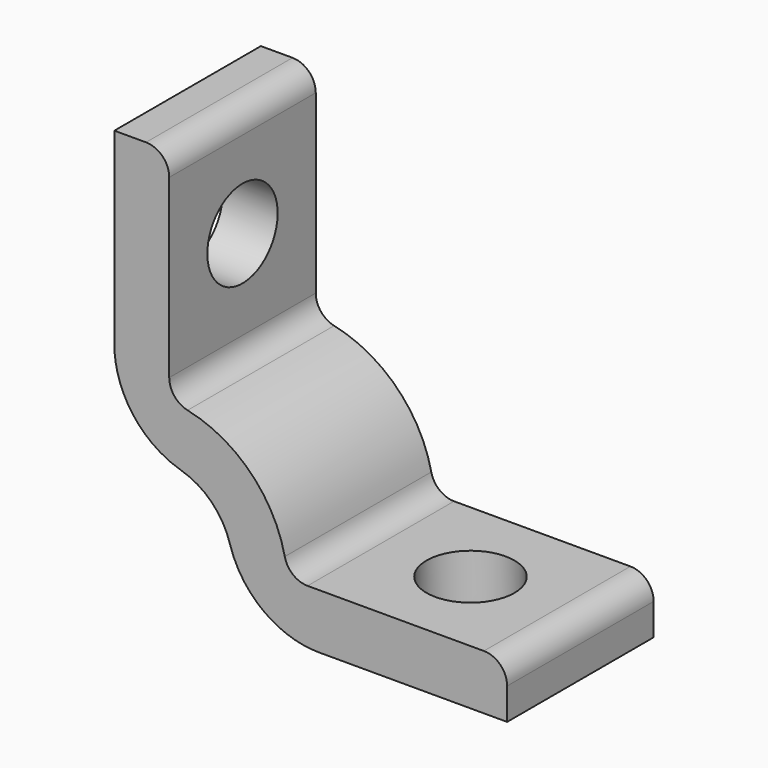
from build123d import *

# Parameters (mm, degrees)
F1_DEPTH = 10
F2_R     = 2.4
F3_DEPTH = 2.9972
F7_R     = 5.08
F8_R     = 1.27


# Not quite as in the source:
# - a pattern or mirror of a feature is missing from the dataset's text; its kind, count and spacing are read off the source's solid


with BuildPart() as f1:
    # F0 (on Front) → F1 (new body)
    with BuildSketch(Plane.XZ):
        with BuildLine():
            ThreePointArc((0, 3.9243), (2.7748991414, 2.7748991414), (3.9243, 0))
            Line((3.9243, 0), (3.9243, -2.54))
            Line((3.9243, -2.54), (18.9063833089, -2.54))
            Line((18.9063833089, -2.54), (18.9063833089, 0.4572))
            Line((18.9063833089, 0.4572), (6.9063833089, 0.4572))
            ThreePointArc((6.9063833089, 0.4572), (4.894239586, 4.894239586), (0.4572, 6.9063833089))
            Line((0.4572, 6.9063833089), (0.4572, 18.9063833089))
            Line((0.4572, 18.9063833089), (-2.54, 18.9063833089))
            Line((-2.54, 18.9063833089), (-2.54, 3.9243))
            Line((-2.54, 3.9243), (0, 3.9243))
        make_face()
    extrude(amount=F1_DEPTH)

    # F2 (on face) → F3 (cut, through all)
    with BuildSketch(Plane.XY.offset(0.4572)):
        with Locations((12.9063833089, -5)):
            Circle(F2_R)
    f3 = extrude(amount=-F3_DEPTH, mode=Mode.SUBTRACT)

    # F3_copies: F3 across plane
    add(f3.mirror(Plane(origin=(0, 0, 0), x_dir=(-0.7071067812, 0, -0.7071067812), z_dir=(-0.7071067812, 0, 0.7071067812))), mode=Mode.SUBTRACT)

    # F7
    f7_edges = [f1.edges().sort_by_distance(p)[0] for p in [
        (-2.54, -5, 3.9243),
        (3.9243, -5, -2.54),
    ]]
    fillet(f7_edges, radius=F7_R)

    # F8
    f8_edges = [f1.edges().sort_by_distance(p)[0] for p in [
        (0.4572, -5, 18.906383),
        (0.4572, -5, 6.906383),
        (6.906383, -5, 0.4572),
        (18.906383, -5, 0.4572),
    ]]
    fillet(f8_edges, radius=F8_R)


solid = f1.part
